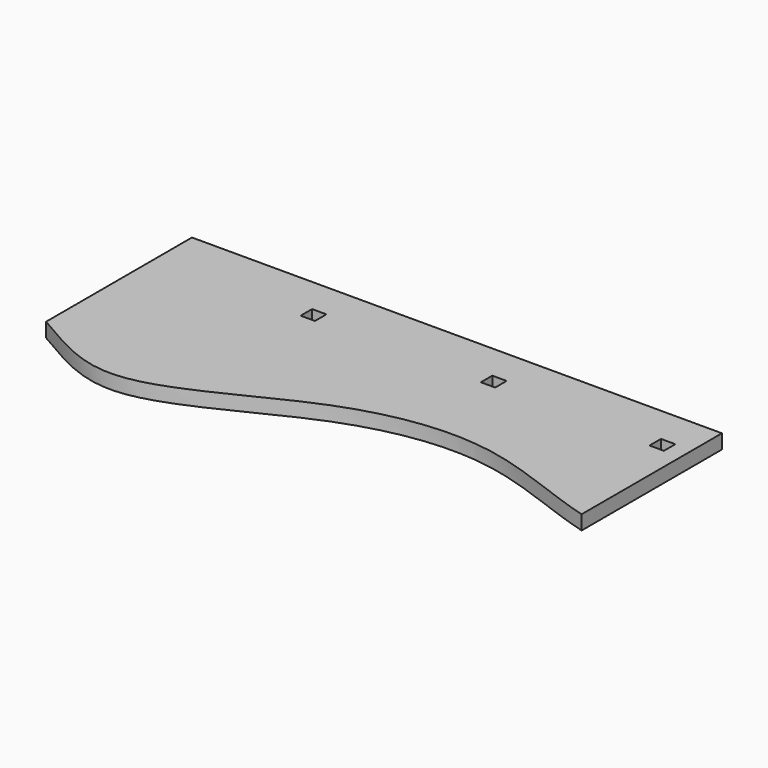
from build123d import *

# Parameters (mm, degrees)
F0_W     = 25.4
F0_H     = 25.4
F1_DEPTH = 25.4


with BuildPart() as f1:
    # F0 (on Top) → F1 (new body)
    with BuildSketch(Plane.XY):
        with BuildLine():
            Line((1377.054914093, 553.4051656723), (818.254914093, 553.4051656723))
            Line((818.254914093, 553.4051656723), (818.254914093, 230.0433814526))
            add(Edge.make_bspline(
                [(818.254914093, 230.0433814526), (869.7513088234, 201.0817050342), (993.6259790946, 113.597779136), (1272.8033875168, 302.84451887), (1538.9749454978, 336.9281412477), (1684.7084265303, 262.9397603077), (1758.054914093, 242.4248605967)],
                knots=[0, 0, 0, 0, 0.215962379, 0.4972360733, 0.7570041226, 1, 1, 1, 1], degree=3))
            Line((1758.054914093, 242.4248605967), (1758.054914093, 553.4051656723))
            Line((1758.054914093, 553.4051656723), (1377.054914093, 553.4051656723))
        make_face()
        with Locations((1094.9438001633, 477.0052220345)):
            Rectangle(F0_W, F0_H, mode=Mode.SUBTRACT)
        with Locations((1414.502778244, 477.0052220345)):
            Rectangle(F0_W, F0_H, mode=Mode.SUBTRACT)
        with Locations((1715.457358551, 474.8164500713)):
            Rectangle(F0_W, F0_H, mode=Mode.SUBTRACT)
    extrude(amount=F1_DEPTH)


solid = f1.part
